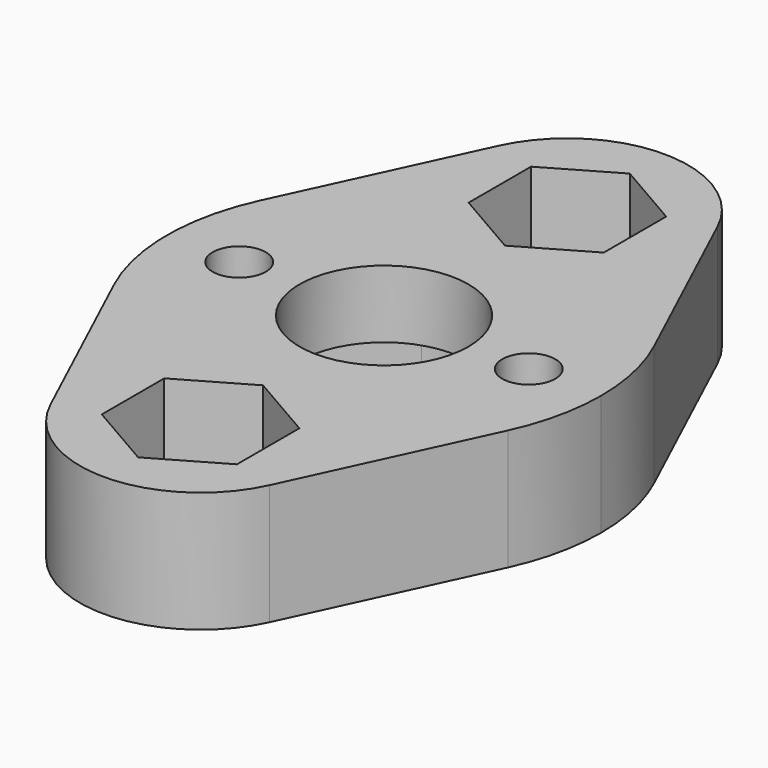
from build123d import *

# Parameters (mm, degrees)
F0_R     = 1.1
F0_R_2   = 3.5
F1_DEPTH = 5
F2_R     = 1.6
F3_DEPTH = 3.9
F5_START = -2.8
F5_DEPTH = 22.2


with BuildPart() as f1:
    # F0 (on Top) → F1 (new body)
    with BuildSketch(Plane.XY):
        with BuildLine():
            ThreePointArc((-1.4743268336, 8.8784210526), (-0.3170781184, 11.0682670266), (1.6, 9.5))
            ThreePointArc((1.6, 9.5), (1.5682670266, 9.1829218816), (1.4743268336, 8.8784210526))
            ThreePointArc((1.4743268336, 8.8784210526), (3.1253325319, 8.4399227819), (4.6637452107, 7.6973684211))
            ThreePointArc((4.6637452107, 7.6973684211), (4.9152174954, 8.5831374295), (5, 9.5))
            ThreePointArc((5, 9.5), (4.882412579, 10.5779830278), (4.5351810367, 11.6052631579))
            ThreePointArc((4.5351810367, 11.6052631579), (0, 14.5), (-4.5351810367, 11.6052631579))
            ThreePointArc((-4.5351810367, 11.6052631579), (-4.9972964036, 9.6644039381), (-4.6637452107, 7.6973684211))
            ThreePointArc((-4.6637452107, 7.6973684211), (-3.1253325319, 8.4399227819), (-1.4743268336, 8.8784210526))
        make_face()
        with BuildLine():
            ThreePointArc((1.4743268336, 8.8784210526), (0, 7.9), (-1.4743268336, 8.8784210526))
            ThreePointArc((-1.4743268336, 8.8784210526), (-3.1253325319, 8.4399227819), (-4.6637452107, 7.6973684211))
            ThreePointArc((-4.6637452107, 7.6973684211), (0, 4.5), (4.6637452107, 7.6973684211))
            ThreePointArc((4.6637452107, 7.6973684211), (3.1253325319, 8.4399227819), (1.4743268336, 8.8784210526))
        make_face()
        with BuildLine():
            ThreePointArc((4.6637452107, 7.6973684211), (0, 4.5), (-4.6637452107, 7.6973684211))
            ThreePointArc((-4.6637452107, 7.6973684211), (-6.7045766773, 6.0040529294), (-8.1633258661, 3.7894736842))
            ThreePointArc((-8.1633258661, 3.7894736842), (-9, 0), (-8.1633258661, -3.7894736842))
            ThreePointArc((-8.1633258661, -3.7894736842), (-6.7045766773, -6.0040529294), (-4.6637452107, -7.6973684211))
            ThreePointArc((-4.6637452107, -7.6973684211), (0, -4.5), (4.6637452107, -7.6973684211))
            ThreePointArc((4.6637452107, -7.6973684211), (6.7045766773, -6.0040529294), (8.1633258661, -3.7894736842))
            ThreePointArc((8.1633258661, -3.7894736842), (8.7883426423, -1.94036945), (9, 0))
            ThreePointArc((9, 0), (8.7883426423, 1.94036945), (8.1633258661, 3.7894736842))
            ThreePointArc((8.1633258661, 3.7894736842), (6.7045766773, 6.0040529294), (4.6637452107, 7.6973684211))
        make_face()
        with Locations((-6, 0)):
            Circle(F0_R, mode=Mode.SUBTRACT)
        Circle(F0_R_2, mode=Mode.SUBTRACT)
        with Locations((6, 0)):
            Circle(F0_R, mode=Mode.SUBTRACT)
        with BuildLine():
            ThreePointArc((-8.1633258661, 3.7894736842), (-6.7045766773, 6.0040529294), (-4.6637452107, 7.6973684211))
            ThreePointArc((-4.6637452107, 7.6973684211), (-4.9972964036, 9.6644039381), (-4.5351810367, 11.6052631579))
            Line((-4.5351810367, 11.6052631579), (-8.1633258661, 3.7894736842))
        make_face()
        with BuildLine():
            ThreePointArc((5, 9.5), (4.9152174954, 8.5831374295), (4.6637452107, 7.6973684211))
            ThreePointArc((4.6637452107, 7.6973684211), (6.7045766773, 6.0040529294), (8.1633258661, 3.7894736842))
            Line((8.1633258661, 3.7894736842), (4.5351810367, 11.6052631579))
            ThreePointArc((4.5351810367, 11.6052631579), (4.882412579, 10.5779830278), (5, 9.5))
        make_face()
        with BuildLine():
            ThreePointArc((-4.6637452107, -7.6973684211), (-6.7045766773, -6.0040529294), (-8.1633258661, -3.7894736842))
            Line((-8.1633258661, -3.7894736842), (-4.5351810367, -11.6052631579))
            ThreePointArc((-4.5351810367, -11.6052631579), (-4.9972964036, -9.6644039381), (-4.6637452107, -7.6973684211))
        make_face()
        with BuildLine():
            ThreePointArc((-1.4743268336, -8.8784210526), (-3.1253325319, -8.4399227819), (-4.6637452107, -7.6973684211))
            ThreePointArc((-4.6637452107, -7.6973684211), (-4.9972964036, -9.6644039381), (-4.5351810367, -11.6052631579))
            ThreePointArc((-4.5351810367, -11.6052631579), (0, -14.5), (4.5351810367, -11.6052631579))
            ThreePointArc((4.5351810367, -11.6052631579), (4.882412579, -10.5779830278), (5, -9.5))
            ThreePointArc((5, -9.5), (4.9152174954, -8.5831374295), (4.6637452107, -7.6973684211))
            ThreePointArc((4.6637452107, -7.6973684211), (3.1253325319, -8.4399227819), (1.4743268336, -8.8784210526))
            ThreePointArc((1.4743268336, -8.8784210526), (1.5682670266, -9.1829218816), (1.6, -9.5))
            ThreePointArc((1.6, -9.5), (-0.3170781184, -11.0682670266), (-1.4743268336, -8.8784210526))
        make_face()
        with BuildLine():
            ThreePointArc((4.6637452107, -7.6973684211), (0, -4.5), (-4.6637452107, -7.6973684211))
            ThreePointArc((-4.6637452107, -7.6973684211), (-3.1253325319, -8.4399227819), (-1.4743268336, -8.8784210526))
            ThreePointArc((-1.4743268336, -8.8784210526), (0, -7.9), (1.4743268336, -8.8784210526))
            ThreePointArc((1.4743268336, -8.8784210526), (3.1253325319, -8.4399227819), (4.6637452107, -7.6973684211))
        make_face()
        with BuildLine():
            Line((4.5351810367, -11.6052631579), (8.1633258661, -3.7894736842))
            ThreePointArc((8.1633258661, -3.7894736842), (6.7045766773, -6.0040529294), (4.6637452107, -7.6973684211))
            ThreePointArc((4.6637452107, -7.6973684211), (4.9152174954, -8.5831374295), (5, -9.5))
            ThreePointArc((5, -9.5), (4.882412579, -10.5779830278), (4.5351810367, -11.6052631579))
        make_face()
    extrude(amount=F1_DEPTH)

    # F2 (on face) → F3 (cut)
    with BuildSketch(Plane.XY.offset(5)):
        Polygon((2.8, 7.8834192463), (2.8, 11.1165807537), (0, 12.7331615075), (-2.8, 11.1165807537), (-2.8, 7.8834192463), (0, 6.2668384925), align=None)
        with Locations((0, 9.5)):
            Circle(F2_R, mode=Mode.SUBTRACT)
        Polygon((-2.8, -11.1165807537), (0, -12.7331615075), (2.8, -11.1165807537), (2.8, -7.8834192463), (0, -6.2668384925), (-2.8, -7.8834192463), align=None)
    extrude(amount=-F3_DEPTH, mode=Mode.SUBTRACT)

    # F4 (on face) → F5 (cut)
    with BuildSketch(Plane.XY.offset(5).offset(F5_START)):
        with BuildLine():
            Line((-1.5033333333, 3.8144447681), (-6.6966666667, 1.7676695267))
            ThreePointArc((-6.6966666667, 1.7676695267), (-7.9, 0), (-6.6966666667, -1.7676695267))
            Line((-6.6966666667, -1.7676695267), (-1.5033333333, -3.8144447681))
            ThreePointArc((-1.5033333333, -3.8144447681), (0, -4.1), (1.5033333333, -3.8144447681))
            Line((1.5033333333, -3.8144447681), (6.6966666667, -1.7676695267))
            ThreePointArc((6.6966666667, -1.7676695267), (7.9, 0), (6.6966666667, 1.7676695267))
            Line((6.6966666667, 1.7676695267), (1.5033333333, 3.8144447681))
            ThreePointArc((1.5033333333, 3.8144447681), (0, 4.1), (-1.5033333333, 3.8144447681))
        make_face()
    extrude(amount=-F5_DEPTH, mode=Mode.SUBTRACT)


solid = f1.part
